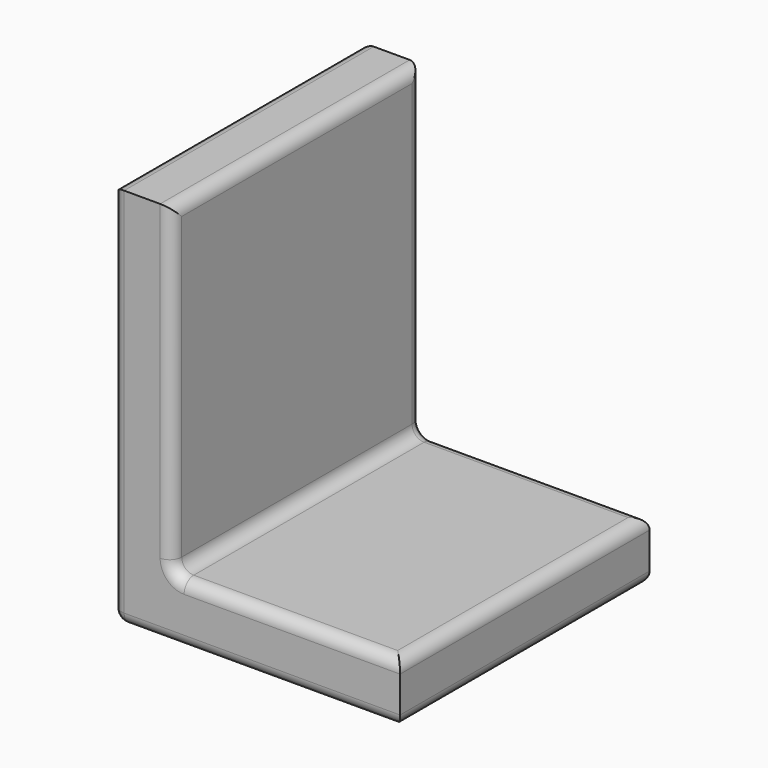
from build123d import *

# Parameters (mm, degrees)
F0_W         = 63.5
F0_H         = 342.9
F0_H_2       = 63.5
F0_W_2       = 241.3
F1_DEPTH     = 165.1
F2_R         = 12.7
F3_R         = 12.7
F4_T1_DEPTH  = 425.45
F4_T3_DEPTH  = 393.7
F4_S7_W      = 12.7
F4_S7_H      = 12.7
F4_T8_DEPTH  = 12.7
F4_S13_W     = 12.7
F4_S13_H     = 12.7
F4_T14_DEPTH = 12.7


# Not quite as in the source:
# - a fillet or chamfer that OpenCascade refuses, or shapes differently, is made with other operations: its cross-section is extruded or revolved along the edge and cut away or added


with BuildPart() as f1:
    # F0 (on Front) → F1 (new body, symmetric)
    with BuildSketch(Plane.XZ):
        with Locations((-120.65, 198.9844056189)):
            Rectangle(F0_W, F0_H)
        with Locations((-120.65, -4.2155943811)):
            Rectangle(F0_W, F0_H_2)
        with Locations((31.75, -4.2155943811)):
            Rectangle(F0_W_2, F0_H_2)
    extrude(amount=F1_DEPTH, both=True)

    # F2
    f2_edges = [f1.edges().sort_by_distance(p)[0] for p in [
        (31.75, -165.1, 27.534406),
        (152.4, 0, 27.534406),
        (31.75, 165.1, 27.534406),
        (-88.9, 0, 27.534406),
        (-88.9, 165.1, 198.984406),
        (-88.9, -165.1, 198.984406),
        (-88.9, 0, 370.434406),
    ]]
    fillet(f2_edges, radius=F2_R)

    # F3
    f3_edges = [f1.edges().sort_by_distance(p)[0] for p in [
        (0, -165.1, -35.965594),
        (152.4, 0, -35.965594),
        (0, 165.1, -35.965594),
        (-152.4, 0, -35.965594),
    ]]
    fillet(f3_edges, radius=F3_R)

    # F4: fillet of radius 12.7 on 3 edges, made by hand

    # F4_s2 → F4_t1 (cut)
    with BuildSketch(Plane.XY.offset(-23.2655943811)):
        with BuildLine():
            ThreePointArc((-152.4, -152.4), (-148.6802561211, -161.3802561211), (-139.7, -165.1))
            Line((-139.7, -165.1), (-152.4, -165.1))
            Line((-152.4, -165.1), (-152.4, -152.4))
        make_face()
        with BuildLine():
            ThreePointArc((-139.7, 165.1), (-148.6802561211, 161.3802561211), (-152.4, 152.4))
            Line((-152.4, 152.4), (-152.4, 165.1))
            Line((-152.4, 165.1), (-139.7, 165.1))
        make_face()
    extrude(amount=F4_T1_DEPTH, mode=Mode.SUBTRACT)

    # F4_s4 → F4_t3 (cut)
    with BuildSketch(Plane.XZ.offset(-196.85)):
        with BuildLine():
            ThreePointArc((-152.4, 357.7344056189), (-148.6802561211, 366.71466174), (-139.7, 370.4344056189))
            Line((-139.7, 370.4344056189), (-152.4, 370.4344056189))
            Line((-152.4, 370.4344056189), (-152.4, 357.7344056189))
        make_face()
    extrude(amount=F4_T3_DEPTH, mode=Mode.SUBTRACT)


with BuildPart() as f4_tool6:
    # F4_s7 → F4_t8 (new body)
    with BuildSketch(Plane.XZ.offset(-152.4)):
        with Locations((-146.05, -29.6155943811)):
            Rectangle(F4_S7_W, F4_S7_H)
    extrude(amount=-F4_T8_DEPTH)

    # F4_s9 → F4_t10 (revolve, cut)
    with BuildSketch(Plane(origin=(-139.7, 152.4, -23.2655943811), x_dir=(0.7071067812, 0, 0.7071067812), z_dir=(-0.7071067812, 0, 0.7071067812))):
        with BuildLine():
            ThreePointArc((0, -12.7), (12.7, 0), (0, 12.7))
            Line((0, 12.7), (0, -12.7))
        make_face()
    revolve(axis=Axis((-139.7, 152.4, -23.2655943811), (0, 1, 0)), mode=Mode.SUBTRACT)


with BuildPart() as f1_1:
    add(f1.part)

    # F4_t5: cut F4_tool6
    add(f4_tool6.part, mode=Mode.SUBTRACT)


with BuildPart() as f4_tool12:
    # F4_s13 → F4_t14 (new body)
    with BuildSketch(Plane.YZ.offset(-139.7)):
        with Locations((-158.75, -29.6155943811)):
            Rectangle(F4_S13_W, F4_S13_H)
    extrude(amount=-F4_T14_DEPTH)

    # F4_s15 → F4_t16 (revolve, cut)
    with BuildSketch(Plane(origin=(-139.7, -152.4, -23.2655943811), x_dir=(0, 0.7071067812, 0.7071067812), z_dir=(0, -0.7071067812, 0.7071067812))):
        with BuildLine():
            ThreePointArc((0, -12.7), (12.7, 0), (0, 12.7))
            Line((0, 12.7), (0, -12.7))
        make_face()
    revolve(axis=Axis((-139.7, -152.4, -23.2655943811), (-1, 0, 0)), mode=Mode.SUBTRACT)


with BuildPart() as f1_2:
    add(f1_1.part)

    # F4_t11: cut F4_tool12
    add(f4_tool12.part, mode=Mode.SUBTRACT)


solid = f1_2.part
